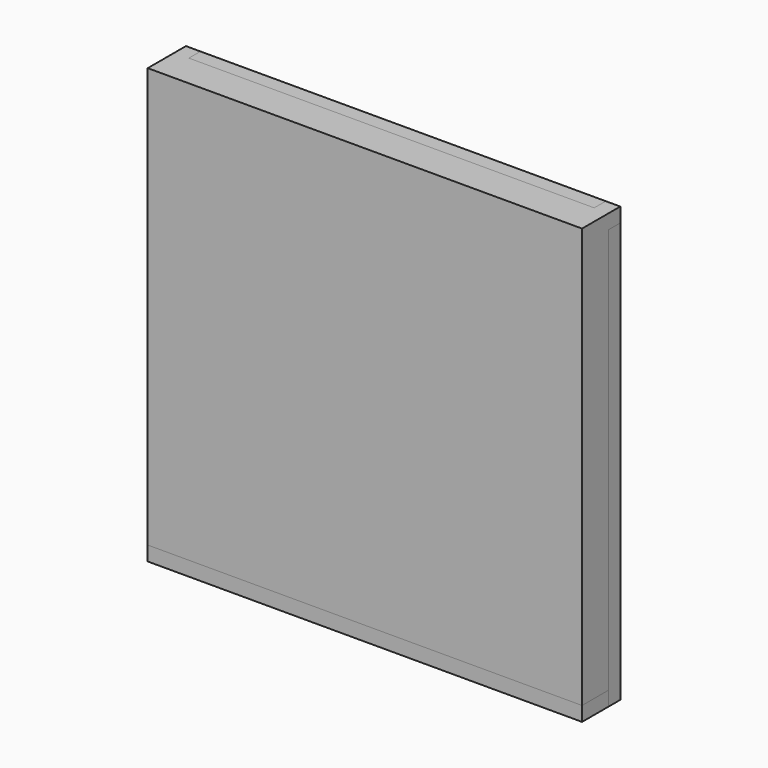
from build123d import *

# Parameters (mm, degrees)
F0_W      = 139.96
F0_H      = 139.96
F0_R      = 7.1
F1_DEPTH  = 3.5
F3_W      = 139.96
F3_H      = 139.96
F4_DEPTH  = 8
F7_DEPTH  = 11.5
F8_W      = 149.96
F8_H      = 5
F9_DEPTH  = 11.5
F10_W     = 5
F10_H     = 5
F11_DEPTH = 5
F13_DEPTH = 5


with BuildPart() as f1:
    # F0 (on Front) → F1 (new body)
    with BuildSketch(Plane.XZ):
        with Locations((-11.0969811678, -6.305641681)):
            Rectangle(F0_W, F0_H)
        with Locations((-61.0969811678, -56.305641681)):
            Circle(F0_R, mode=Mode.SUBTRACT)
        with Locations((-36.0969811678, -56.305641681)):
            Circle(F0_R, mode=Mode.SUBTRACT)
        with Locations((-61.0969811678, -31.305641681)):
            Circle(F0_R, mode=Mode.SUBTRACT)
        with Locations((-36.0969811678, -31.305641681)):
            Circle(F0_R, mode=Mode.SUBTRACT)
        with Locations((-11.0969811678, -56.305641681)):
            Circle(F0_R, mode=Mode.SUBTRACT)
        with Locations((13.9030188322, -56.305641681)):
            Circle(F0_R, mode=Mode.SUBTRACT)
        with Locations((38.9030188322, -56.305641681)):
            Circle(F0_R, mode=Mode.SUBTRACT)
        with Locations((-11.0969811678, -31.305641681)):
            Circle(F0_R, mode=Mode.SUBTRACT)
        with Locations((13.9030188322, -31.305641681)):
            Circle(F0_R, mode=Mode.SUBTRACT)
        with Locations((38.9030188322, -31.305641681)):
            Circle(F0_R, mode=Mode.SUBTRACT)
        with Locations((-61.0969811678, -6.305641681)):
            Circle(F0_R, mode=Mode.SUBTRACT)
        with Locations((-61.0969811678, 18.694358319)):
            Circle(F0_R, mode=Mode.SUBTRACT)
        with Locations((-36.0969811678, -6.305641681)):
            Circle(F0_R, mode=Mode.SUBTRACT)
        with Locations((-36.0969811678, 18.694358319)):
            Circle(F0_R, mode=Mode.SUBTRACT)
        with Locations((-61.0969811678, 43.694358319)):
            Circle(F0_R, mode=Mode.SUBTRACT)
        with Locations((-36.0969811678, 43.694358319)):
            Circle(F0_R, mode=Mode.SUBTRACT)
        with Locations((-11.0969811678, -6.305641681)):
            Circle(F0_R, mode=Mode.SUBTRACT)
        with Locations((13.9030188322, -6.305641681)):
            Circle(F0_R, mode=Mode.SUBTRACT)
        with Locations((-11.0969811678, 18.694358319)):
            Circle(F0_R, mode=Mode.SUBTRACT)
        with Locations((13.9030188322, 18.694358319)):
            Circle(F0_R, mode=Mode.SUBTRACT)
        with Locations((38.9030188322, -6.305641681)):
            Circle(F0_R, mode=Mode.SUBTRACT)
        with Locations((38.9030188322, 18.694358319)):
            Circle(F0_R, mode=Mode.SUBTRACT)
        with Locations((-11.0969811678, 43.694358319)):
            Circle(F0_R, mode=Mode.SUBTRACT)
        with Locations((13.9030188322, 43.694358319)):
            Circle(F0_R, mode=Mode.SUBTRACT)
        with Locations((38.9030188322, 43.694358319)):
            Circle(F0_R, mode=Mode.SUBTRACT)
    extrude(amount=F1_DEPTH)

    # F8 (on Front) → F9 (join)
    with BuildSketch(Plane.XZ):
        with Locations((-11.0969811678, -78.785641681)):
            Rectangle(F8_W, F8_H)
    extrude(amount=F9_DEPTH)


with BuildPart() as f4:
    # F3 (on offset) → F4 (new body)
    with BuildSketch(Plane.XZ.offset(3.5)):
        with Locations((-11.0969811678, -6.305641681)):
            Rectangle(F3_W, F3_H)
    extrude(amount=F4_DEPTH)

    # F6 (on offset) → F7 (join)
    with BuildSketch(Plane.XZ.offset(11.5)):
        Polygon((-81.0769811678, -76.285641681), (-81.0769811678, 63.674358319), (58.8830188322, 63.674358319), (58.8830188322, -76.285641681), (63.8830188322, -76.285641681), (63.8830188322, 68.674358319), (-86.0769811678, 68.674358319), (-86.0769811678, -76.285641681), align=None)
    extrude(amount=-F7_DEPTH)

    # F10 (on Front) → F11 (join)
    with BuildSketch(Plane.XZ):
        with Locations((-83.5769811678, 66.174358319)):
            Rectangle(F10_W, F10_H)
        with Locations((61.3830188322, 66.174358319)):
            Rectangle(F10_W, F10_H)
    extrude(amount=-F11_DEPTH)


with BuildPart() as f13:
    # F12 (on Front) → F13 (new body)
    with BuildSketch(Plane.XZ):
        Polygon((58.8830188322, 63.674358319), (58.8830188322, 68.674358319), (-81.0769811678, 68.674358319), (-81.0769811678, 63.674358319), (-86.0769811678, 63.674358319), (-86.0769811678, -81.285641681), (63.8830188322, -81.285641681), (63.8830188322, 63.674358319), align=None)
    extrude(amount=-F13_DEPTH)


solid = Compound([f1.part, f4.part, f13.part])
